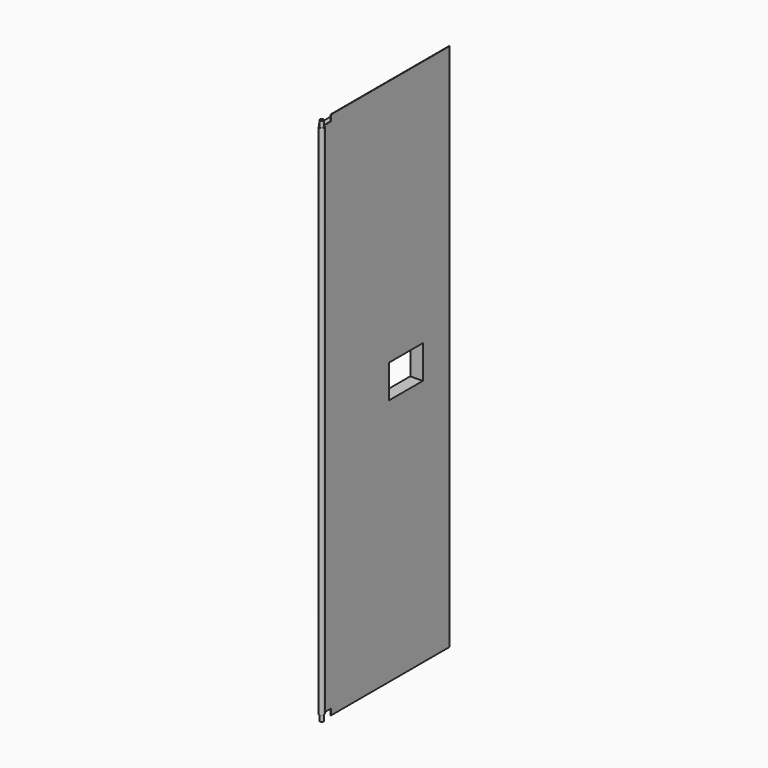
from build123d import *

# Parameters (mm, degrees)
F1_DEPTH       = 0.889
F2_W           = 304.8
F2_H           = 1060.45
F3_DEPTH       = 25.4
F5_DEPTH       = 317.501
F7_DEPTH       = 1085.851
F8_R           = 1.27
F9_W           = 88.9
F9_H           = 34.925
F10_DEPTH      = 26.29
F11_R          = 5.03555
F11_R_2        = 3.96875
F12_DEPTH      = 542.925
F12_DEPTH_BACK = 542.925
F13_R          = 3.96875
F14_DEPTH      = 555.625
F14_DEPTH_BACK = 555.625


# Not quite as in the source:
# - a feature names something its author has since deleted; it is built from what else it names


with BuildPart() as f1:
    # F0 (on Right) → F1 (new body)
    with BuildSketch(Plane.YZ):
        Polygon((165.1, 555.625), (-146.05, 555.625), (-146.05, 542.925), (-165.1, 542.925), (-165.1, 0), (165.1, 0), align=None)
        Polygon((165.1, -555.625), (165.1, 0), (-165.1, 0), (-165.1, -542.925), (-146.05, -542.925), (-146.05, -555.625), align=None)
    extrude(amount=-F1_DEPTH)

    # F2 (on face) → F3 (join)
    with BuildSketch(Plane(origin=(-0.889, 0, 0), x_dir=(0, -1, 0), z_dir=(-1, 0, 0))):
        Rectangle(F2_W, F2_H)
    extrude(amount=F3_DEPTH)

    # F4 (on face) → F5 (cut, through all)
    with BuildSketch(Plane(origin=(0, 152.4, 0), x_dir=(-1, 0, 0), z_dir=(0, 1, 0))):
        Polygon((2.1336, -530.225), (26.289, -530.225), (2.1336, -492.9112069626), align=None)
        Polygon((2.1336, 492.9112069626), (26.289, 530.225), (2.1336, 530.225), align=None)
    extrude(amount=-F5_DEPTH, mode=Mode.SUBTRACT)

    # F6 (on face) → F7 (cut, through all)
    with BuildSketch(Plane.XY.offset(530.225)):
        Polygon((-2.1336, -152.4), (-2.1336, -127.550815087), (-38.989, -152.4), align=None)
        Polygon((-2.1336, 152.4), (-26.289, 152.4), (-2.1336, 115.0862069626), align=None)
    extrude(amount=-F7_DEPTH, mode=Mode.SUBTRACT)

    # F8
    f8_edges = [f1.edges().sort_by_distance(p)[0] for p in [
        (-2.1336, -6.232304, 492.911207),
        (-2.1336, -6.232304, -492.911207),
    ]]
    fillet(f8_edges, radius=F8_R)

    # F9 (on face) → F10 (cut, through all)
    with BuildSketch(Plane.YZ):
        with Locations((50.8, 17.4625)):
            Rectangle(F9_W, F9_H)
        with Locations((50.8, -17.4625)):
            Rectangle(F9_W, F9_H)
    extrude(amount=-F10_DEPTH, mode=Mode.SUBTRACT)


with BuildPart() as f12:
    # F11 (on Top) → F12 (new body, two sides)
    with BuildSketch(Plane.XY) as f12_sk:
        with Locations((0, -170.13555)):
            Circle(F11_R)
        with Locations((0, -170.13555)):
            Circle(F11_R_2, mode=Mode.SUBTRACT)
    extrude(amount=F12_DEPTH)
    extrude(f12_sk.sketch, amount=-F12_DEPTH_BACK)

    # F13 (on Top) → F14 (join, two sides)
    with BuildSketch(Plane.XY) as f14_sk:
        with Locations((0, -170.13555)):
            Circle(F13_R)
    extrude(amount=F14_DEPTH)
    extrude(f14_sk.sketch, amount=-F14_DEPTH_BACK)


solid = Compound([f1.part, f12.part])
